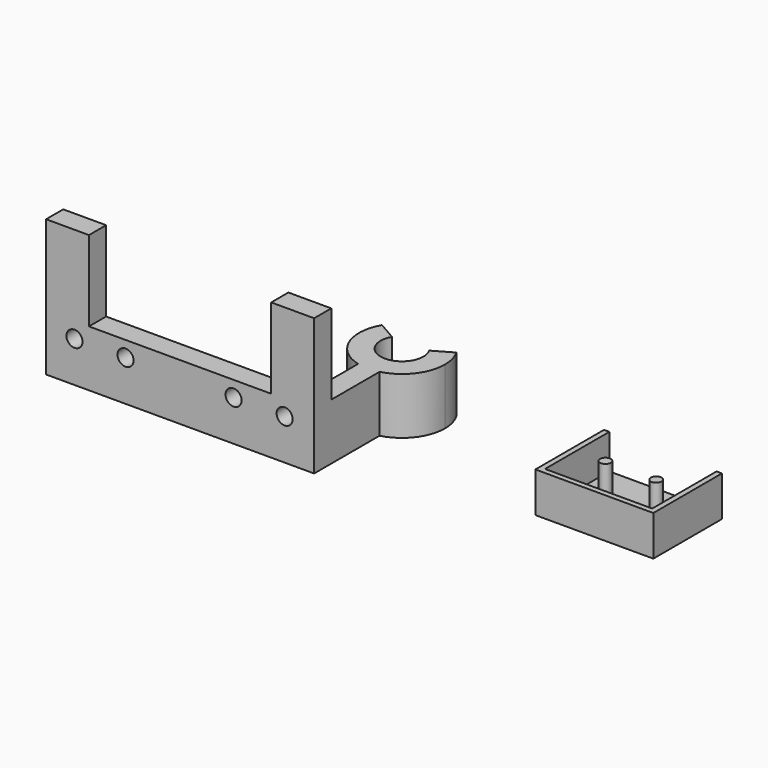
from build123d import *

# Parameters (mm, degrees)
F0_W      = 22
F0_H      = 16
F1_DEPTH  = 7.5
F2_W      = 20
F2_H      = 15
F3_DEPTH  = 6.5
F5_DEPTH  = 6.5
F7_DEPTH  = 10.5
F9_W      = 8
F9_H      = 4
F10_DEPTH = 15
F12_D     = 3
F12_DEPTH = 10
F12_TIP   = 0.9012909285


# Not quite as in the source:
# - a feature names something its author has since deleted; it is built from what else it names


with BuildPart() as f1:
    # F0 (on Top) → F1 (new body)
    with BuildSketch(Plane.XY):
        with Locations((11, 8)):
            Rectangle(F0_W, F0_H)
    extrude(amount=F1_DEPTH)

    # F2 (on face) → F3 (cut)
    with BuildSketch(Plane.XY.offset(7.5)):
        with Locations((11, 8.5)):
            Rectangle(F2_W, F2_H)
    extrude(amount=-F3_DEPTH, mode=Mode.SUBTRACT)

    # F4 (on face) → F5 (join)
    with BuildSketch(Plane.XY.offset(1)):
        with BuildLine():
            ThreePointArc((5.275, 8.5), (6.275, 7.5), (7.275, 8.5))
            Line((7.275, 8.5), (5.275, 8.5))
        make_face()
        with BuildLine():
            Line((5.275, 8.5), (7.275, 8.5))
            ThreePointArc((7.275, 8.5), (6.275, 9.5), (5.275, 8.5))
        make_face()
        with BuildLine():
            ThreePointArc((16.725, 8.5), (15.725, 9.5), (14.725, 8.5))
            Line((14.725, 8.5), (16.725, 8.5))
        make_face()
        with BuildLine():
            Line((16.725, 8.5), (14.725, 8.5))
            ThreePointArc((14.725, 8.5), (15.725, 7.5), (16.725, 8.5))
        make_face()
    extrude(amount=F5_DEPTH)


with BuildPart() as f7:
    # F6 (on Top) → F7 (new body)
    with BuildSketch(Plane.XY):
        with BuildLine():
            Line((0.0722974215, 15.1097724214), (-3.3918041936, 17.1097724214))
            ThreePointArc((-3.3918041936, 17.1097724214), (-3.8406014795, 10.0146369826), (1.5363990366, 5.363805729))
            Line((1.5363990366, 5.363805729), (1.5363990366, 9.1097724214))
            Line((1.5363990366, 9.1097724214), (3.5363990366, 9.1097724214))
            ThreePointArc((3.5363990366, 9.1097724214), (0.0722974215, 11.1097724214), (0.0722974215, 15.1097724214))
        make_face()
        with BuildLine():
            ThreePointArc((3.5363990366, 5.1097724214), (4.5444333765, 5.1735348513), (5.5363990366, 5.363805729))
            Line((5.5363990366, 5.363805729), (5.5363990366, 9.1097724214))
            Line((5.5363990366, 9.1097724214), (3.5363990366, 9.1097724214))
            Line((3.5363990366, 9.1097724214), (3.5363990366, 5.1097724214))
        make_face()
        with BuildLine():
            ThreePointArc((1.5363990366, 5.363805729), (2.5283646968, 5.1735348513), (3.5363990366, 5.1097724214))
            Line((3.5363990366, 5.1097724214), (3.5363990366, 9.1097724214))
            Line((3.5363990366, 9.1097724214), (1.5363990366, 9.1097724214))
            Line((1.5363990366, 9.1097724214), (1.5363990366, 5.363805729))
        make_face()
        with BuildLine():
            ThreePointArc((5.5363990366, 5.363805729), (9.860954357, 8.2107929359), (11.5363990366, 13.1097724214))
            ThreePointArc((11.5363990366, 13.1097724214), (11.263805647, 15.1803247822), (10.4646022669, 17.1097724214))
            Line((10.4646022669, 17.1097724214), (7.0005006518, 15.1097724214))
            ThreePointArc((7.0005006518, 15.1097724214), (7.4001023418, 14.1450486018), (7.5363990366, 13.1097724214))
            ThreePointArc((7.5363990366, 13.1097724214), (6.3648261614, 10.2813452967), (3.5363990366, 9.1097724214))
            Line((3.5363990366, 9.1097724214), (5.5363990366, 9.1097724214))
            Line((5.5363990366, 9.1097724214), (5.5363990366, 5.363805729))
        make_face()
        with BuildLine():
            Line((5.5363990366, -5.8902275786), (5.5363990366, 5.363805729))
            ThreePointArc((5.5363990366, 5.363805729), (4.5444333765, 5.1735348513), (3.5363990366, 5.1097724214))
            Line((3.5363990366, 5.1097724214), (3.5363990366, -5.8902275786))
            Line((3.5363990366, -5.8902275786), (5.5363990366, -5.8902275786))
        make_face()
        with BuildLine():
            Line((3.5363990366, -5.8902275786), (3.5363990366, 5.1097724214))
            ThreePointArc((3.5363990366, 5.1097724214), (2.5283646968, 5.1735348513), (1.5363990366, 5.363805729))
            Line((1.5363990366, 5.363805729), (1.5363990366, -5.8902275786))
            Line((1.5363990366, -5.8902275786), (3.5363990366, -5.8902275786))
        make_face()
        Polygon((5.5363990366, -9.8902275786), (5.5363990366, -5.8902275786), (3.5363990366, -5.8902275786), (1.5363990366, -5.8902275786), (-44.4636009634, -5.8902275786), (-44.4636009634, -9.8902275786), align=None)
    extrude(amount=F7_DEPTH)


with BuildPart() as f7_1:
    # F8: moved
    add(f7.part.moved(Location((-38.9, 0, 0))))

    # F9 (on face) → F10 (join)
    with BuildSketch(Plane.XY.offset(10.5)):
        with Locations((-37.3636009634, -7.8902275786)):
            Rectangle(F9_W, F9_H)
        with Locations((-79.3636009634, -7.8902275786)):
            Rectangle(F9_W, F9_H)
    extrude(amount=F10_DEPTH)

    # F12
    with Locations(Plane.XZ.offset(9.8902275786)):
        with Locations((-78.0636009634, 7.6), (-68.5386009634, 7.6), (-48.3886009634, 7.6), (-38.8636009634, 7.6)):
            Hole(F12_D / 2, depth=F12_DEPTH)
            with Locations((0, 0, -(F12_DEPTH + F12_TIP / 2))):  # 118° drill point
                Cone(0, F12_D / 2, F12_TIP, mode=Mode.SUBTRACT)


solid = Compound([f1.part, f7_1.part])
